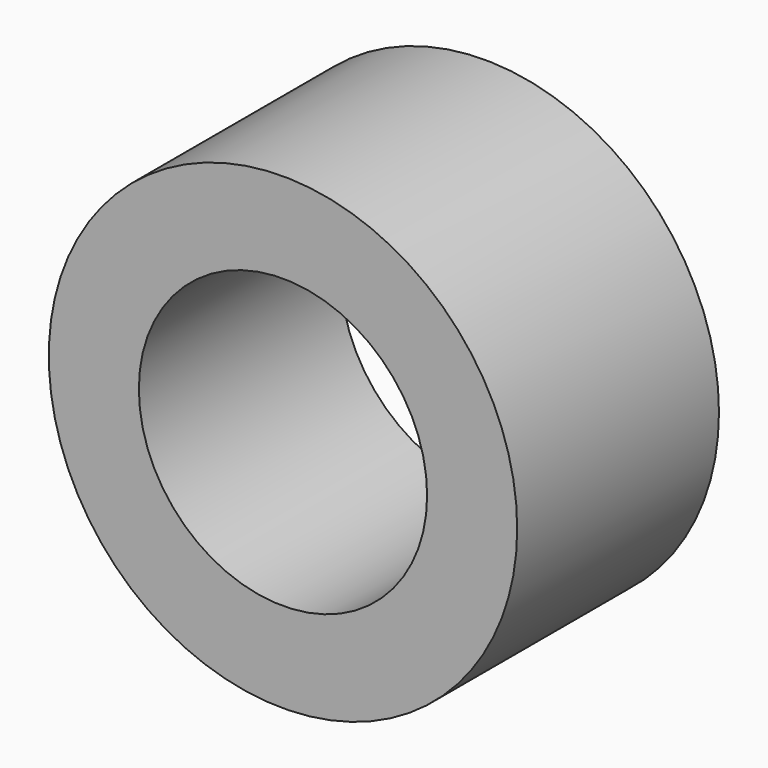
from build123d import *

# Parameters (mm, degrees)
F0_R     = 32.5
F0_R_2   = 20
F1_DEPTH = 17.5


# Not quite as in the source:
# - the program builds the solid bodies; features that only make, move or delete a surface that nothing else refers to are left out


with BuildPart() as f1:
    # F0 (on Front) → F1 (new body, symmetric)
    with BuildSketch(Plane.XZ):
        Circle(F0_R)
        Circle(F0_R_2, mode=Mode.SUBTRACT)
    extrude(amount=F1_DEPTH, both=True)


solid = f1.part
